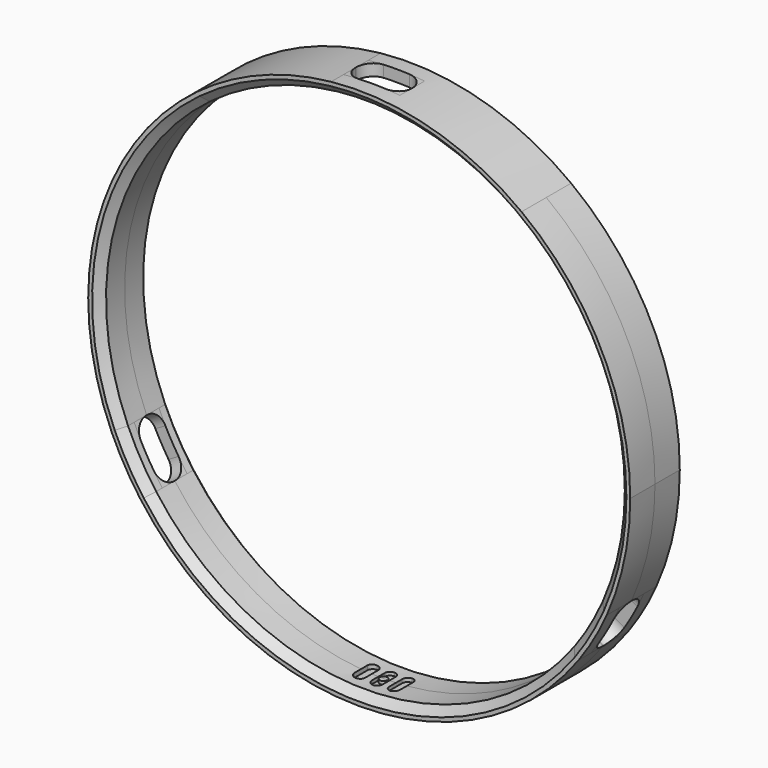
from build123d import *

# Parameters (mm, degrees)
F1_DEPTH      = 4
F1_DEPTH_BACK = 4
F2_SIZE       = 1
F4_DEPTH      = 2
F4_DEPTH_BACK = 2
F5_T4_DEPTH   = 11.2085158977
F5_S5_R       = 33.5
F5_T6_DEPTH   = 8
F5_S7_R       = 35
F5_T8_DEPTH   = 8
F5_T12_DEPTH  = 11.2085158977
F5_S13_R      = 35
F5_T14_DEPTH  = 8
F5_S15_R      = 33.5
F5_T16_DEPTH  = 8
F5_T20_DEPTH  = 11.2085158977
F5_S21_R      = 33.5
F5_T22_DEPTH  = 8
F5_S23_R      = 35
F5_T24_DEPTH  = 8
F5_T28_DEPTH  = 11.2085158977
F5_S29_R      = 33.5
F5_T30_DEPTH  = 8
F5_S31_R      = 35
F5_T32_DEPTH  = 8
F5_T36_DEPTH  = 11.2085158977
F5_S37_R      = 33.5
F5_T38_DEPTH  = 8
F5_S39_R      = 35
F5_T40_DEPTH  = 8
F5_T44_DEPTH  = 11.2085158977
F5_S45_R      = 33.5
F5_T46_DEPTH  = 8
F5_S47_R      = 35
F5_T48_DEPTH  = 8
F5_T52_DEPTH  = 11.2085158977
F5_S53_R      = 33.5
F5_T54_DEPTH  = 8
F5_S55_R      = 35
F5_T56_DEPTH  = 8
F5_T60_DEPTH  = 11.2085158977
F5_S61_R      = 33.5
F5_T62_DEPTH  = 8
F5_S63_R      = 35
F5_T64_DEPTH  = 8
F5_T68_DEPTH  = 11.2085158977
F5_S69_R      = 33.5
F5_T70_DEPTH  = 7
F5_S71_R      = 35
F5_T72_DEPTH  = 7
F5_T76_DEPTH  = 11.2085158977
F5_S77_R      = 33.5
F5_T78_DEPTH  = 7
F5_S79_R      = 35
F5_T80_DEPTH  = 7
F5_T84_DEPTH  = 11.2085158977
F5_S85_R      = 33.5
F5_T86_DEPTH  = 7
F5_S87_R      = 35
F5_T88_DEPTH  = 7
F5_T92_DEPTH  = 11.2085158977
F5_S93_R      = 33.5
F5_T94_DEPTH  = 7
F5_S95_R      = 35
F5_T96_DEPTH  = 7
F6_R          = 0.5
F7_DEPTH      = 33.93


# Not quite as in the source:
# - a fillet or chamfer that OpenCascade refuses, or shapes differently, is made with other operations: its cross-section is extruded or revolved along the edge and cut away or added


with BuildPart() as f1:
    # F0 (on Front) → F1 (new body, two sides)
    with BuildSketch(Plane.XZ) as f1_sk:
        with BuildLine():
            ThreePointArc((3.6332620451, 33.3023934112), (12.2794013905, 31.1683541672), (20.057750608, 26.8316350703))
            Line((20.057750608, 26.8316350703), (20.9639415908, 28.0270075637))
            ThreePointArc((20.9639415908, 28.0270075637), (12.7577794854, 32.5920091833), (3.6332620451, 34.8109093089))
            Line((3.6332620451, 34.8109093089), (3.6332620451, 33.3023934112))
        make_face()
        with BuildLine():
            ThreePointArc((-3.6332620451, 33.3023934112), (0, 33.5), (3.6332620451, 33.3023934112))
            Line((3.6332620451, 33.3023934112), (3.6332620451, 34.8109093089))
            ThreePointArc((3.6332620451, 34.8109093089), (0, 35), (-3.6332620451, 34.8109093089))
            Line((-3.6332620451, 34.8109093089), (-3.6332620451, 33.3023934112))
        make_face()
        with BuildLine():
            ThreePointArc((-20.057750608, 26.8316350703), (-12.2794013905, 31.1683541672), (-3.6332620451, 33.3023934112))
            Line((-3.6332620451, 33.3023934112), (-3.6332620451, 34.8109093089))
            ThreePointArc((-3.6332620451, 34.8109093089), (-12.7577794854, 32.5920091833), (-20.9639415908, 28.0270075637))
            Line((-20.9639415908, 28.0270075637), (-20.057750608, 26.8316350703))
        make_face()
        with BuildLine():
            ThreePointArc((-30.6573497234, -13.504699476), (-32.4000049624, 8.5140870583), (-20.057750608, 26.8316350703))
            Line((-20.057750608, 26.8316350703), (-20.9639415908, 28.0270075637))
            ThreePointArc((-20.9639415908, 28.0270075637), (-33.8727203235, 8.8112892295), (-31.9637628129, -14.2589574248))
            Line((-31.9637628129, -14.2589574248), (-30.6573497234, -13.504699476))
        make_face()
        with BuildLine():
            Line((-28.3305007678, -20.5519518841), (-27.0240876784, -19.7976939352))
            ThreePointArc((-27.0240876784, -19.7976939352), (-29.0118510268, -16.75), (-30.6573497234, -13.504699476))
            Line((-30.6573497234, -13.504699476), (-31.9637628129, -14.2589574248))
            ThreePointArc((-31.9637628129, -14.2589574248), (-30.3108891325, -17.5), (-28.3305007678, -20.5519518841))
        make_face()
        with BuildLine():
            Line((28.3305007678, -20.5519518841), (27.0240876784, -19.7976939352))
            ThreePointArc((27.0240876784, -19.7976939352), (0, -33.5), (-27.0240876784, -19.7976939352))
            Line((-27.0240876784, -19.7976939352), (-28.3305007678, -20.5519518841))
            ThreePointArc((-28.3305007678, -20.5519518841), (0, -35), (28.3305007678, -20.5519518841))
        make_face()
        with BuildLine():
            Line((31.9637628129, -14.2589574248), (30.6573497234, -13.504699476))
            ThreePointArc((30.6573497234, -13.504699476), (29.0118510268, -16.75), (27.0240876784, -19.7976939352))
            Line((27.0240876784, -19.7976939352), (28.3305007678, -20.5519518841))
            ThreePointArc((28.3305007678, -20.5519518841), (30.3108891325, -17.5), (31.9637628129, -14.2589574248))
        make_face()
        with BuildLine():
            ThreePointArc((20.057750608, 26.8316350703), (29.9514995064, 15.00525499), (33.5, 0))
            ThreePointArc((33.5, 0), (32.7816352226, -6.9003182631), (30.6573497234, -13.504699476))
            Line((30.6573497234, -13.504699476), (31.9637628129, -14.2589574248))
            ThreePointArc((31.9637628129, -14.2589574248), (34.2325261882, -7.2893175795), (35, 0))
            ThreePointArc((35, 0), (31.2948714303, 15.6726201434), (20.9639415908, 28.0270075637))
            Line((20.9639415908, 28.0270075637), (20.057750608, 26.8316350703))
        make_face()
        with BuildLine():
            Line((28.3305007678, -20.5519518841), (27.0240876784, -19.7976939352))
            ThreePointArc((27.0240876784, -19.7976939352), (0, -33.5), (-27.0240876784, -19.7976939352))
            Line((-27.0240876784, -19.7976939352), (-28.3305007678, -20.5519518841))
            ThreePointArc((-28.3305007678, -20.5519518841), (0, -35), (28.3305007678, -20.5519518841))
        make_face()
        with BuildLine():
            ThreePointArc((20.057750608, 26.8316350703), (29.9514995064, 15.00525499), (33.5, 0))
            ThreePointArc((33.5, 0), (32.7816352226, -6.9003182631), (30.6573497234, -13.504699476))
            Line((30.6573497234, -13.504699476), (31.9637628129, -14.2589574248))
            ThreePointArc((31.9637628129, -14.2589574248), (34.2325261882, -7.2893175795), (35, 0))
            ThreePointArc((35, 0), (31.2948714303, 15.6726201434), (20.9639415908, 28.0270075637))
            Line((20.9639415908, 28.0270075637), (20.057750608, 26.8316350703))
        make_face()
        with BuildLine():
            ThreePointArc((-30.6573497234, -13.504699476), (-32.4000049624, 8.5140870583), (-20.057750608, 26.8316350703))
            Line((-20.057750608, 26.8316350703), (-20.9639415908, 28.0270075637))
            ThreePointArc((-20.9639415908, 28.0270075637), (-33.8727203235, 8.8112892295), (-31.9637628129, -14.2589574248))
            Line((-31.9637628129, -14.2589574248), (-30.6573497234, -13.504699476))
        make_face()
        with BuildLine():
            Line((28.3305007678, -20.5519518841), (27.0240876784, -19.7976939352))
            ThreePointArc((27.0240876784, -19.7976939352), (0, -33.5), (-27.0240876784, -19.7976939352))
            Line((-27.0240876784, -19.7976939352), (-28.3305007678, -20.5519518841))
            ThreePointArc((-28.3305007678, -20.5519518841), (0, -35), (28.3305007678, -20.5519518841))
        make_face()
    extrude(amount=F1_DEPTH)
    extrude(f1_sk.sketch, amount=-F1_DEPTH_BACK)

    # F2
    f2_edges = [f1.edges().sort_by_distance(p)[0] for p in [
        (-30.65735, -4, 13.504699),
        (-30.65735, 4, 13.504699),
    ]]
    chamfer(f2_edges, length=F2_SIZE)

    # F0 (on Front) → F4 (cut, two sides)
    with BuildSketch(Plane.XZ) as f4_sk:
        with BuildLine():
            ThreePointArc((-3.6332620451, 34.8109093089), (0, 35), (3.6332620451, 34.8109093089))
            Line((3.6332620451, 34.8109093089), (3.6332620451, 36.968215256))
            Line((3.6332620451, 36.968215256), (-3.6332620451, 36.968215256))
            Line((-3.6332620451, 36.968215256), (-3.6332620451, 34.8109093089))
        make_face()
        with BuildLine():
            ThreePointArc((-3.6332620451, 33.3023934112), (0, 33.5), (3.6332620451, 33.3023934112))
            Line((3.6332620451, 33.3023934112), (3.6332620451, 34.8109093089))
            ThreePointArc((3.6332620451, 34.8109093089), (0, 35), (-3.6332620451, 34.8109093089))
            Line((-3.6332620451, 34.8109093089), (-3.6332620451, 33.3023934112))
        make_face()
        with BuildLine():
            Line((3.6332620451, 31.6989157826), (3.6332620451, 33.3023934112))
            ThreePointArc((3.6332620451, 33.3023934112), (0, 33.5), (-3.6332620451, 33.3023934112))
            Line((-3.6332620451, 33.3023934112), (-3.6332620451, 31.6989157826))
            Line((-3.6332620451, 31.6989157826), (3.6332620451, 31.6989157826))
        make_face()
        with BuildLine():
            ThreePointArc((27.0240876784, -19.7976939352), (29.0118510268, -16.75), (30.6573497234, -13.504699476))
            Line((30.6573497234, -13.504699476), (7.2665240901, 0))
            Line((7.2665240901, 0), (3.3491878185, -6.1289841281))
            Line((3.3491878185, -6.1289841281), (27.0240876784, -19.7976939352))
        make_face()
        with BuildLine():
            Line((31.9637628129, -14.2589574248), (30.6573497234, -13.504699476))
            ThreePointArc((30.6573497234, -13.504699476), (29.0118510268, -16.75), (27.0240876784, -19.7976939352))
            Line((27.0240876784, -19.7976939352), (28.3305007678, -20.5519518841))
            ThreePointArc((28.3305007678, -20.5519518841), (30.3108891325, -17.5), (31.9637628129, -14.2589574248))
        make_face()
        with BuildLine():
            Line((33.8320445668, -15.3376103984), (31.9637628129, -14.2589574248))
            ThreePointArc((31.9637628129, -14.2589574248), (30.3108891325, -17.5), (28.3305007678, -20.5519518841))
            Line((28.3305007678, -20.5519518841), (30.1987825217, -21.6306048576))
            Line((30.1987825217, -21.6306048576), (33.8320445668, -15.3376103984))
        make_face()
        with BuildLine():
            ThreePointArc((-30.6573497234, -13.504699476), (-29.0118510268, -16.75), (-27.0240876784, -19.7976939352))
            Line((-27.0240876784, -19.7976939352), (-3.2841431884, -6.0914305934))
            Line((-3.2841431884, -6.0914305934), (-6.8559292529, 0.2370570398))
            Line((-6.8559292529, 0.2370570398), (-30.6573497234, -13.504699476))
        make_face()
        with BuildLine():
            Line((-30.1987825217, -21.6306048576), (-28.3305007678, -20.5519518841))
            ThreePointArc((-28.3305007678, -20.5519518841), (-30.3108891325, -17.5), (-31.9637628129, -14.2589574248))
            Line((-31.9637628129, -14.2589574248), (-33.8320445668, -15.3376103984))
            Line((-33.8320445668, -15.3376103984), (-30.1987825217, -21.6306048576))
        make_face()
        with BuildLine():
            Line((-28.3305007678, -20.5519518841), (-27.0240876784, -19.7976939352))
            ThreePointArc((-27.0240876784, -19.7976939352), (-29.0118510268, -16.75), (-30.6573497234, -13.504699476))
            Line((-30.6573497234, -13.504699476), (-31.9637628129, -14.2589574248))
            ThreePointArc((-31.9637628129, -14.2589574248), (-30.3108891325, -17.5), (-28.3305007678, -20.5519518841))
        make_face()
    extrude(amount=-F4_DEPTH, mode=Mode.SUBTRACT)
    extrude(f4_sk.sketch, amount=F4_DEPTH_BACK, mode=Mode.SUBTRACT)

    # F5: fillet of radius 1.94 on 12 edges, made by hand


with BuildPart() as f5_tool2:
    # F5_s3 → F5_t4 (new body)
    with BuildSketch(Plane(origin=(24.6404954925, 0, -14.2261967056), x_dir=(0, 1, 0), z_dir=(0.8660254038, 0, -0.5))):
        with BuildLine():
            ThreePointArc((0.06, -3.6332620451), (1.4317871555, -3.0650492006), (2, -1.6932620451))
            Line((2, -1.6932620451), (2, -3.6332620451))
            Line((2, -3.6332620451), (0.06, -3.6332620451))
        make_face()
    extrude(amount=F5_T4_DEPTH)

    # F5_s5 → F5_t6 (cut, symmetric)
    with BuildSketch(Plane.XZ.offset(-1)):
        Circle(F5_S5_R)
    extrude(amount=F5_T6_DEPTH, both=True, mode=Mode.SUBTRACT)

    # F5_s7 → F5_t8 (intersect, symmetric)
    with BuildSketch(Plane.XZ.offset(-1)):
        Circle(F5_S7_R)
    extrude(amount=F5_T8_DEPTH, both=True, mode=Mode.INTERSECT)


with BuildPart() as f1_1:
    add(f1.part)

    # F5_t1: union F5_tool2
    add(f5_tool2.part)


with BuildPart() as f5_tool10:
    # F5_s11 → F5_t12 (new body)
    with BuildSketch(Plane(origin=(34.3473549987, 0, -19.8304546544), x_dir=(0, 1, 0), z_dir=(-0.8660254038, 0, 0.5))):
        with BuildLine():
            ThreePointArc((0.06, -3.6332620451), (1.4317871555, -3.0650492006), (2, -1.6932620451))
            Line((2, -1.6932620451), (2, -3.6332620451))
            Line((2, -3.6332620451), (0.06, -3.6332620451))
        make_face()
    extrude(amount=F5_T12_DEPTH)

    # F5_s13 → F5_t14 (intersect, symmetric)
    with BuildSketch(Plane.XZ.offset(-1)):
        Circle(F5_S13_R)
    extrude(amount=F5_T14_DEPTH, both=True, mode=Mode.INTERSECT)

    # F5_s15 → F5_t16 (cut, symmetric)
    with BuildSketch(Plane.XZ.offset(-1)):
        Circle(F5_S15_R)
    extrude(amount=F5_T16_DEPTH, both=True, mode=Mode.SUBTRACT)


with BuildPart() as f1_2:
    add(f1_1.part)

    # F5_t9: union F5_tool10
    add(f5_tool10.part)


with BuildPart() as f5_tool18:
    # F5_s19 → F5_t20 (new body)
    with BuildSketch(Plane(origin=(34.3473549987, 0, -19.8304546544), x_dir=(0, 1, 0), z_dir=(-0.8660254038, 0, 0.5))):
        with BuildLine():
            ThreePointArc((-0.06, -3.6332620451), (-1.4317871555, -3.0650492006), (-2, -1.6932620451))
            Line((-2, -1.6932620451), (-2, -3.6332620451))
            Line((-2, -3.6332620451), (-0.06, -3.6332620451))
        make_face()
    extrude(amount=F5_T20_DEPTH)

    # F5_s21 → F5_t22 (cut, symmetric)
    with BuildSketch(Plane.XZ.offset(1)):
        Circle(F5_S21_R)
    extrude(amount=F5_T22_DEPTH, both=True, mode=Mode.SUBTRACT)

    # F5_s23 → F5_t24 (intersect, symmetric)
    with BuildSketch(Plane.XZ.offset(1)):
        Circle(F5_S23_R)
    extrude(amount=F5_T24_DEPTH, both=True, mode=Mode.INTERSECT)


with BuildPart() as f1_3:
    add(f1_2.part)

    # F5_t17: union F5_tool18
    add(f5_tool18.part)


with BuildPart() as f5_tool26:
    # F5_s27 → F5_t28 (new body)
    with BuildSketch(Plane(origin=(24.6404954925, 0, -14.2261967056), x_dir=(0, 1, 0), z_dir=(0.8660254038, 0, -0.5))):
        with BuildLine():
            ThreePointArc((-2, -1.6932620451), (-1.4317871555, -3.0650492006), (-0.06, -3.6332620451))
            Line((-0.06, -3.6332620451), (-2, -3.6332620451))
            Line((-2, -3.6332620451), (-2, -1.6932620451))
        make_face()
    extrude(amount=F5_T28_DEPTH)

    # F5_s29 → F5_t30 (cut, symmetric)
    with BuildSketch(Plane.XZ.offset(1)):
        Circle(F5_S29_R)
    extrude(amount=F5_T30_DEPTH, both=True, mode=Mode.SUBTRACT)

    # F5_s31 → F5_t32 (intersect, symmetric)
    with BuildSketch(Plane.XZ.offset(1)):
        Circle(F5_S31_R)
    extrude(amount=F5_T32_DEPTH, both=True, mode=Mode.INTERSECT)


with BuildPart() as f1_4:
    add(f1_3.part)

    # F5_t25: union F5_tool26
    add(f5_tool26.part)


with BuildPart() as f5_tool34:
    # F5_s35 → F5_t36 (new body)
    with BuildSketch(Plane(origin=(-34.3473549987, 0, -19.8304546544), x_dir=(0, 1, 0), z_dir=(0.8660254038, 0, 0.5))):
        with BuildLine():
            ThreePointArc((0.06, -3.6332620451), (1.4317871555, -3.0650492006), (2, -1.6932620451))
            Line((2, -1.6932620451), (2, -3.6332620451))
            Line((2, -3.6332620451), (0.06, -3.6332620451))
        make_face()
    extrude(amount=F5_T36_DEPTH)

    # F5_s37 → F5_t38 (cut, symmetric)
    with BuildSketch(Plane.XZ.offset(-1)):
        Circle(F5_S37_R)
    extrude(amount=F5_T38_DEPTH, both=True, mode=Mode.SUBTRACT)

    # F5_s39 → F5_t40 (intersect, symmetric)
    with BuildSketch(Plane.XZ.offset(-1)):
        Circle(F5_S39_R)
    extrude(amount=F5_T40_DEPTH, both=True, mode=Mode.INTERSECT)


with BuildPart() as f1_5:
    add(f1_4.part)

    # F5_t33: union F5_tool34
    add(f5_tool34.part)


with BuildPart() as f5_tool42:
    # F5_s43 → F5_t44 (new body)
    with BuildSketch(Plane(origin=(-24.6404954925, 0, -14.2261967056), x_dir=(0, 1, 0), z_dir=(-0.8660254038, 0, -0.5))):
        with BuildLine():
            ThreePointArc((0.06, -3.6332620451), (1.4317871555, -3.0650492006), (2, -1.6932620451))
            Line((2, -1.6932620451), (2, -3.6332620451))
            Line((2, -3.6332620451), (0.06, -3.6332620451))
        make_face()
    extrude(amount=F5_T44_DEPTH)

    # F5_s45 → F5_t46 (cut, symmetric)
    with BuildSketch(Plane.XZ.offset(-1)):
        Circle(F5_S45_R)
    extrude(amount=F5_T46_DEPTH, both=True, mode=Mode.SUBTRACT)

    # F5_s47 → F5_t48 (intersect, symmetric)
    with BuildSketch(Plane.XZ.offset(-1)):
        Circle(F5_S47_R)
    extrude(amount=F5_T48_DEPTH, both=True, mode=Mode.INTERSECT)


with BuildPart() as f1_6:
    add(f1_5.part)

    # F5_t41: union F5_tool42
    add(f5_tool42.part)


with BuildPart() as f5_tool50:
    # F5_s51 → F5_t52 (new body)
    with BuildSketch(Plane(origin=(-24.6404954925, 0, -14.2261967056), x_dir=(0, 1, 0), z_dir=(-0.8660254038, 0, -0.5))):
        with BuildLine():
            ThreePointArc((-2, -1.6932620451), (-1.4317871555, -3.0650492006), (-0.06, -3.6332620451))
            Line((-0.06, -3.6332620451), (-2, -3.6332620451))
            Line((-2, -3.6332620451), (-2, -1.6932620451))
        make_face()
    extrude(amount=F5_T52_DEPTH)

    # F5_s53 → F5_t54 (cut, symmetric)
    with BuildSketch(Plane.XZ.offset(1)):
        Circle(F5_S53_R)
    extrude(amount=F5_T54_DEPTH, both=True, mode=Mode.SUBTRACT)

    # F5_s55 → F5_t56 (intersect, symmetric)
    with BuildSketch(Plane.XZ.offset(1)):
        Circle(F5_S55_R)
    extrude(amount=F5_T56_DEPTH, both=True, mode=Mode.INTERSECT)


with BuildPart() as f1_7:
    add(f1_6.part)

    # F5_t49: union F5_tool50
    add(f5_tool50.part)


with BuildPart() as f5_tool58:
    # F5_s59 → F5_t60 (new body)
    with BuildSketch(Plane(origin=(-34.3473549987, 0, -19.8304546544), x_dir=(0, 1, 0), z_dir=(0.8660254038, 0, 0.5))):
        with BuildLine():
            ThreePointArc((-0.06, -3.6332620451), (-1.4317871555, -3.0650492006), (-2, -1.6932620451))
            Line((-2, -1.6932620451), (-2, -3.6332620451))
            Line((-2, -3.6332620451), (-0.06, -3.6332620451))
        make_face()
    extrude(amount=F5_T60_DEPTH)

    # F5_s61 → F5_t62 (cut, symmetric)
    with BuildSketch(Plane.XZ.offset(1)):
        Circle(F5_S61_R)
    extrude(amount=F5_T62_DEPTH, both=True, mode=Mode.SUBTRACT)

    # F5_s63 → F5_t64 (intersect, symmetric)
    with BuildSketch(Plane.XZ.offset(1)):
        Circle(F5_S63_R)
    extrude(amount=F5_T64_DEPTH, both=True, mode=Mode.INTERSECT)


with BuildPart() as f1_8:
    add(f1_7.part)

    # F5_t57: union F5_tool58
    add(f5_tool58.part)


with BuildPart() as f5_tool66:
    # F5_s67 → F5_t68 (new body)
    with BuildSketch(Plane.XY.offset(39.6609093089)):
        with BuildLine():
            ThreePointArc((-3.6332620451, 0.06), (-3.0650492006, 1.4317871555), (-1.6932620451, 2))
            Line((-1.6932620451, 2), (-3.6332620451, 2))
            Line((-3.6332620451, 2), (-3.6332620451, 0.06))
        make_face()
    extrude(amount=-F5_T68_DEPTH)

    # F5_s69 → F5_t70 (cut, symmetric)
    with BuildSketch(Plane.XZ.offset(-1)):
        Circle(F5_S69_R)
    extrude(amount=F5_T70_DEPTH, both=True, mode=Mode.SUBTRACT)

    # F5_s71 → F5_t72 (intersect, symmetric)
    with BuildSketch(Plane.XZ.offset(-1)):
        Circle(F5_S71_R)
    extrude(amount=F5_T72_DEPTH, both=True, mode=Mode.INTERSECT)


with BuildPart() as f1_9:
    add(f1_8.part)

    # F5_t65: union F5_tool66
    add(f5_tool66.part)


with BuildPart() as f5_tool74:
    # F5_s75 → F5_t76 (new body)
    with BuildSketch(Plane.XY.offset(28.4523934112)):
        with BuildLine():
            ThreePointArc((3.6332620451, 0.06), (3.0650492006, 1.4317871555), (1.6932620451, 2))
            Line((1.6932620451, 2), (3.6332620451, 2))
            Line((3.6332620451, 2), (3.6332620451, 0.06))
        make_face()
    extrude(amount=F5_T76_DEPTH)

    # F5_s77 → F5_t78 (cut, symmetric)
    with BuildSketch(Plane.XZ.offset(-1)):
        Circle(F5_S77_R)
    extrude(amount=F5_T78_DEPTH, both=True, mode=Mode.SUBTRACT)

    # F5_s79 → F5_t80 (intersect, symmetric)
    with BuildSketch(Plane.XZ.offset(-1)):
        Circle(F5_S79_R)
    extrude(amount=F5_T80_DEPTH, both=True, mode=Mode.INTERSECT)


with BuildPart() as f1_10:
    add(f1_9.part)

    # F5_t73: union F5_tool74
    add(f5_tool74.part)


with BuildPart() as f5_tool82:
    # F5_s83 → F5_t84 (new body)
    with BuildSketch(Plane.XY.offset(39.6609093089)):
        with BuildLine():
            ThreePointArc((-3.6332620451, -0.06), (-3.0650492006, -1.4317871555), (-1.6932620451, -2))
            Line((-1.6932620451, -2), (-3.6332620451, -2))
            Line((-3.6332620451, -2), (-3.6332620451, -0.06))
        make_face()
    extrude(amount=-F5_T84_DEPTH)

    # F5_s85 → F5_t86 (cut, symmetric)
    with BuildSketch(Plane.XZ.offset(1)):
        Circle(F5_S85_R)
    extrude(amount=F5_T86_DEPTH, both=True, mode=Mode.SUBTRACT)

    # F5_s87 → F5_t88 (intersect, symmetric)
    with BuildSketch(Plane.XZ.offset(1)):
        Circle(F5_S87_R)
    extrude(amount=F5_T88_DEPTH, both=True, mode=Mode.INTERSECT)


with BuildPart() as f1_11:
    add(f1_10.part)

    # F5_t81: union F5_tool82
    add(f5_tool82.part)


with BuildPart() as f5_tool90:
    # F5_s91 → F5_t92 (new body)
    with BuildSketch(Plane.XY.offset(28.4523934112)):
        with BuildLine():
            ThreePointArc((1.6932620451, -2), (3.0650492006, -1.4317871555), (3.6332620451, -0.06))
            Line((3.6332620451, -0.06), (3.6332620451, -2))
            Line((3.6332620451, -2), (1.6932620451, -2))
        make_face()
    extrude(amount=F5_T92_DEPTH)

    # F5_s93 → F5_t94 (cut, symmetric)
    with BuildSketch(Plane.XZ.offset(1)):
        Circle(F5_S93_R)
    extrude(amount=F5_T94_DEPTH, both=True, mode=Mode.SUBTRACT)

    # F5_s95 → F5_t96 (intersect, symmetric)
    with BuildSketch(Plane.XZ.offset(1)):
        Circle(F5_S95_R)
    extrude(amount=F5_T96_DEPTH, both=True, mode=Mode.INTERSECT)


with BuildPart() as f1_12:
    add(f1_11.part)

    # F5_t89: union F5_tool90
    add(f5_tool90.part)

    # F6 (on Top) → F7 (cut)
    with BuildSketch(Plane.XY):
        with BuildLine():
            ThreePointArc((-2.266085241, 1.7133431449), (-2.7610599878, 1.5083178917), (-2.966085241, 1.0133431449))
            Line((-2.966085241, 1.0133431449), (-2.966085241, -1.0790815327))
            ThreePointArc((-2.966085241, -1.0790815327), (-2.7610599878, -1.5740562796), (-2.266085241, -1.7790815327))
            ThreePointArc((-2.266085241, -1.7790815327), (-1.7711104942, -1.5740562796), (-1.566085241, -1.0790815327))
            Line((-1.566085241, -1.0790815327), (-1.566085241, 1.0133431449))
            ThreePointArc((-1.566085241, 1.0133431449), (-1.7711104942, 1.5083178917), (-2.266085241, 1.7133431449))
        make_face()
        with BuildLine():
            ThreePointArc((-0.0126359519, 1.7133431449), (-0.5076106987, 1.5083178917), (-0.7126359519, 1.0133431449))
            Line((-0.7126359519, 1.0133431449), (-0.7126359519, -1.0790815327))
            ThreePointArc((-0.7126359519, -1.0790815327), (-0.5076106987, -1.5740562796), (-0.0126359519, -1.7790815327))
            ThreePointArc((-0.0126359519, -1.7790815327), (0.482338795, -1.5740562796), (0.6873640481, -1.0790815327))
            Line((0.6873640481, -1.0790815327), (0.6873640481, 1.0133431449))
            ThreePointArc((0.6873640481, 1.0133431449), (0.482338795, 1.5083178917), (-0.0126359519, 1.7133431449))
        make_face()
        with Locations((-0.0146476336, -0.0376115397)):
            Circle(F6_R, mode=Mode.SUBTRACT)
        with BuildLine():
            ThreePointArc((2.2403640481, 1.7133431449), (1.7453893013, 1.5083178917), (1.5403640481, 1.0133431449))
            Line((1.5403640481, 1.0133431449), (1.5403640481, -1.0790815327))
            ThreePointArc((1.5403640481, -1.0790815327), (1.7453893013, -1.5740562796), (2.2403640481, -1.7790815327))
            ThreePointArc((2.2403640481, -1.7790815327), (2.735338795, -1.5740562796), (2.9403640481, -1.0790815327))
            Line((2.9403640481, -1.0790815327), (2.9403640481, 1.0133431449))
            ThreePointArc((2.9403640481, 1.0133431449), (2.735338795, 1.5083178917), (2.2403640481, 1.7133431449))
        make_face()
    extrude(amount=-F7_DEPTH, mode=Mode.SUBTRACT)


solid = f1_12.part
